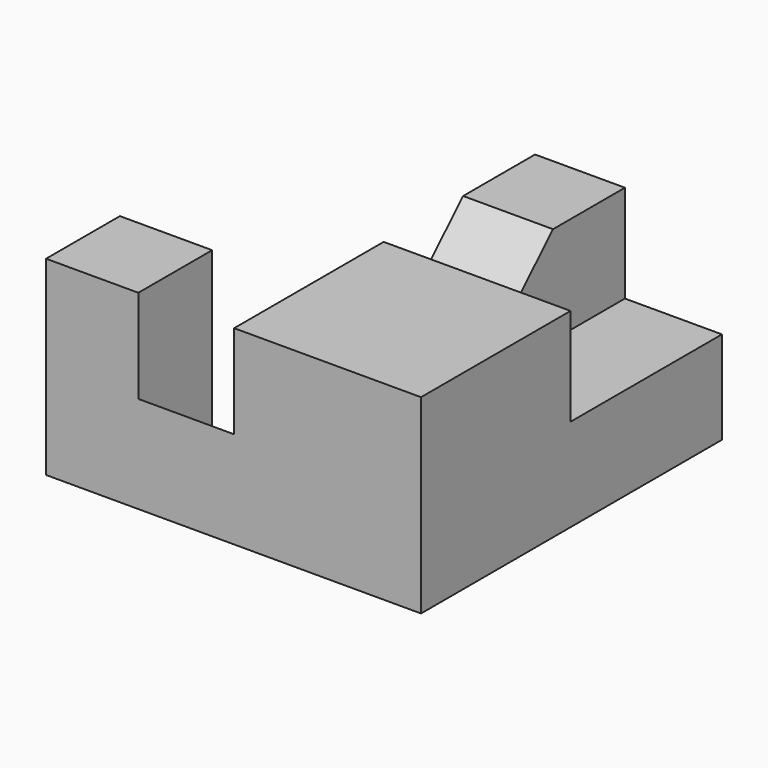
from build123d import *

# Parameters (mm, degrees)
F0_W      = 15.8
F0_H      = 15.8
F1_DEPTH  = 16.1
F3_DEPTH  = 8.1
F5_DEPTH  = 7.8
F6_W      = 15.8
F6_H      = 16
F7_DEPTH  = 7.85
F8_W      = 7.6
F8_H      = 7.6
F9_DEPTH  = 8.25
F11_DEPTH = 7.6


with BuildPart() as f1:
    # F0 (on Top) → F1 (new body)
    with BuildSketch(Plane.XY):
        with Locations((-0.699278047, -1.1891025347)):
            Rectangle(F0_W, F0_H)
    extrude(amount=F1_DEPTH)

    # F2 (on face) → F3 (join)
    with BuildSketch(Plane(origin=(-8.599278047, 0, 0), x_dir=(0, -1, 0), z_dir=(-1, 0, 0))):
        Polygon((1.2891025347, 0), (9.0891025347, 0), (9.0891025347, 8.2), align=None)
    extrude(amount=F3_DEPTH)

    # F4 (on face) → F5 (join)
    with BuildSketch(Plane(origin=(-16.699278047, 0, 0), x_dir=(0, -1, 0), z_dir=(-1, 0, 0))):
        Polygon((1.2891025347, 16.1), (1.2891025347, 0), (9.0891025347, 8.2), (9.0891025347, 16.1), align=None)
        Polygon((1.2891025347, 0), (9.0891025347, 0), (9.0891025347, 8.2), align=None)
    extrude(amount=F5_DEPTH)

    # F6 (on face) → F7 (join)
    with BuildSketch(Plane(origin=(0, 0, 0), x_dir=(1, 0, 0), z_dir=(0, 0, -1))):
        with Locations((-0.699278047, -14.7108974653)):
            Rectangle(F6_W, F6_H)
    extrude(amount=-F7_DEPTH)

    # F8 (on face) → F9 (join, through all)
    with BuildSketch(Plane.XY.offset(7.85)):
        with Locations((-4.799278047, 18.9108974653)):
            Rectangle(F8_W, F8_H)
    extrude(amount=F9_DEPTH)

    # F10 (on face) → F11 (join, through all)
    with BuildSketch(Plane(origin=(-8.599278047, 0, 0), x_dir=(0, -1, 0), z_dir=(-1, 0, 0))):
        Polygon((-6.7108974653, 7.85), (-15.1108974653, 16.1), (-15.1108974653, 7.85), align=None)
    extrude(amount=-F11_DEPTH)


solid = f1.part
